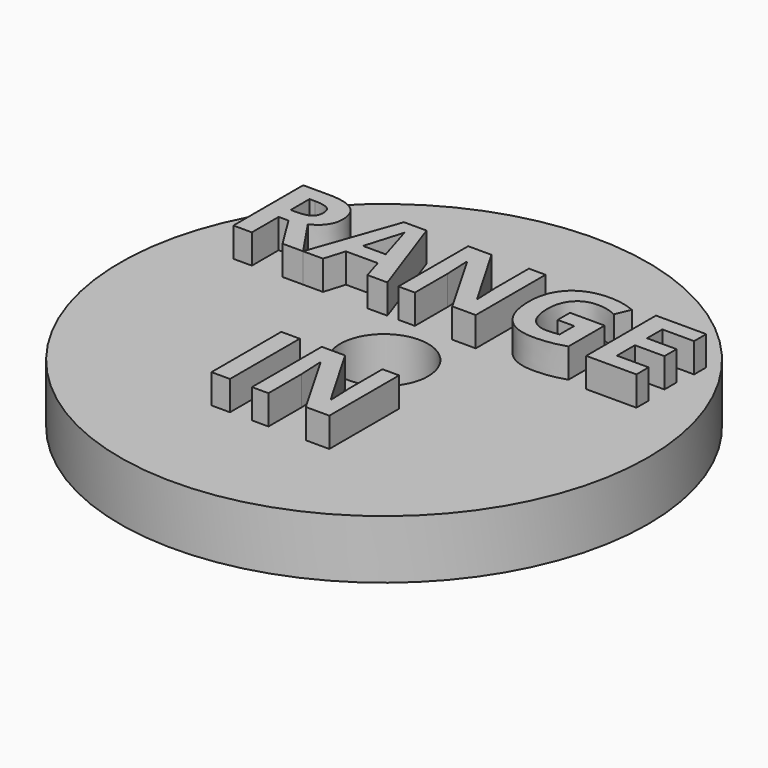
from build123d import *

# Parameters (mm, degrees)
F0_R         = 9
F1_DEPTH     = 2
F2_R         = 1.5
F3_DEPTH     = 2
F4_TEXT_SIZE = 4.1666666667
F5_DEPTH     = 1


# Not quite as in the source:
# - Text() gives the source's letters only with a copy of the font that has no kerning and outlines rounded to 1/6400 em; it was checked with that copy


with BuildPart() as f1:
    # F0 (on Top) → F1 (new body)
    with BuildSketch(Plane.XY):
        with Locations((-42.4070470035, -34.6393212676)):
            Circle(F0_R)
    extrude(amount=F1_DEPTH)

    # F2 (on face) → F3 (cut)
    with BuildSketch(Plane.XY.offset(2)):
        with Locations((-42.4070470035, -34.6393212676)):
            Circle(F2_R)
    extrude(amount=-F3_DEPTH, mode=Mode.SUBTRACT)


with BuildPart() as f5:
    # F4 (on face) → F5 (new body)
    with BuildSketch(Plane.XY.offset(2)):
        with Locations((-49.5616224209, -32.5878109249)):
            Text('RANGE', F4_TEXT_SIZE, font='Open Sans', font_style=FontStyle.BOLD, text_align=(TextAlign.LEFT, TextAlign.BOTTOM))
        with Locations((-44.7354521826, -39.5535393357)):
            Text('IN', F4_TEXT_SIZE, font='Open Sans', font_style=FontStyle.BOLD, text_align=(TextAlign.LEFT, TextAlign.BOTTOM))
    extrude(amount=F5_DEPTH)


solid = Compound([f1.part, f5.part])
